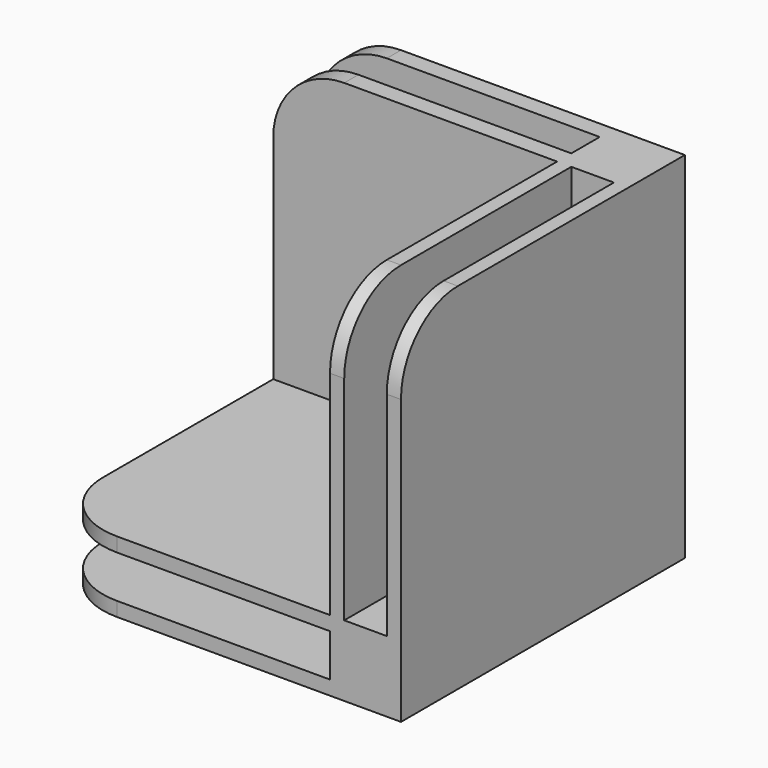
from build123d import *

# Parameters (mm, degrees)
F1_DEPTH = 10
F3_DEPTH = 10
F5_DEPTH = 10
F6_W     = 20
F6_H     = 6
F6_W_2   = 6
F6_H_2   = 30
F6_H_3   = 20
F7_DEPTH = 40
F8_W     = 30
F8_H     = 5
F8_W_2   = 20
F9_DEPTH = 50.001


# Not quite as in the source:
# - a feature names something its author has since deleted; it is built from what else it names


with BuildPart() as f1:
    # F0 (on Top) → F1 (new body)
    with BuildSketch(Plane.XY):
        with BuildLine():
            Line((0, -50), (0, 0))
            Line((0, 0), (-50, 0))
            Line((-50, 0), (-50, -40))
            ThreePointArc((-50, -40), (-47.0710678119, -47.0710678119), (-40, -50))
            Line((-40, -50), (0, -50))
        make_face()
    extrude(amount=F1_DEPTH)

    # F2 (on Right) → F3 (join)
    with BuildSketch(Plane.YZ):
        with BuildLine():
            Line((-50, 10), (0, 10))
            Line((0, 10), (0, 50))
            Line((0, 50), (-40, 50))
            ThreePointArc((-40, 50), (-47.0710678119, 47.0710678119), (-50, 40))
            Line((-50, 40), (-50, 10))
        make_face()
    extrude(amount=-F3_DEPTH)

    # F4 (on Front) → F5 (join)
    with BuildSketch(Plane.XZ):
        with BuildLine():
            Line((-50, 10), (-10, 10))
            Line((-10, 10), (-10, 50))
            Line((-10, 50), (-40, 50))
            ThreePointArc((-40, 50), (-47.0710678119, 47.0710678119), (-50, 40))
            Line((-50, 40), (-50, 10))
        make_face()
    extrude(amount=F5_DEPTH)

    # F6 (on face) → F7 (cut)
    with BuildSketch(Plane.XZ.offset(50)):
        Polygon((-15, 2), (-10, 2), (-10, 8), (-40, 8), (-40, 2), align=None)
        with Locations((-50, 5)):
            Rectangle(F6_W, F6_H)
        with Locations((-5, 25)):
            Rectangle(F6_W_2, F6_H_2)
        with Locations((-5, 50)):
            Rectangle(F6_W_2, F6_H_3)
    extrude(amount=-F7_DEPTH, mode=Mode.SUBTRACT)

    # F8 (on face) → F9 (cut, through all)
    with BuildSketch(Plane.XY.offset(50)):
        with Locations((-25, -5)):
            Rectangle(F8_W, F8_H)
        with Locations((-50, -5)):
            Rectangle(F8_W_2, F8_H)
    extrude(amount=-F9_DEPTH, mode=Mode.SUBTRACT)


solid = f1.part
